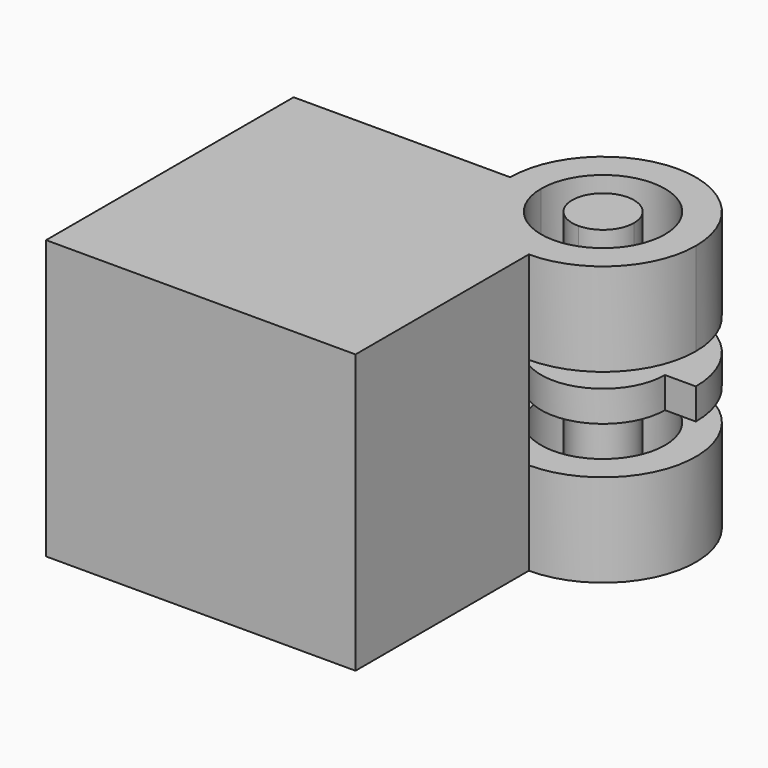
from build123d import *

# Parameters (mm, degrees)
F1_DEPTH  = 3
F2_DEPTH  = 1
F3_DEPTH  = 1
F5_DEPTH  = 1
F6_DEPTH  = 1
F8_DEPTH  = 1
F7_R      = 1
F9_DEPTH  = 1
F11_DEPTH = 3
F12_R     = 2
F13_DEPTH = 3
F14_DEPTH = 3


with BuildPart() as f1:
    # F0 (on Top) → F1 (new body)
    with BuildSketch(Plane.XY):
        with BuildLine():
            Line((-48.9987007827, 31.2983999767), (-55.9987007827, 31.2983999767))
            Line((-55.9987007827, 31.2983999767), (-55.9987007827, 21.2983999767))
            Line((-55.9987007827, 21.2983999767), (-45.9987007827, 21.2983999767))
            Line((-45.9987007827, 21.2983999767), (-45.9987007827, 28.2983999767))
            ThreePointArc((-45.9987007827, 28.2983999767), (-48.1200211262, 29.1770796331), (-48.9987007827, 31.2983999767))
        make_face()
        with BuildLine():
            ThreePointArc((-42.9987007827, 31.2983999767), (-45.9987007827, 34.2983999767), (-48.9987007827, 31.2983999767))
            Line((-48.9987007827, 31.2983999767), (-47.9987007827, 31.2983999767))
            ThreePointArc((-47.9987007827, 31.2983999767), (-45.9987007827, 33.2983999767), (-43.9987007827, 31.2983999767))
            ThreePointArc((-43.9987007827, 31.2983999767), (-44.5844872203, 29.8841864143), (-45.9987007827, 29.2983999767))
            Line((-45.9987007827, 29.2983999767), (-45.9987007827, 28.2983999767))
            ThreePointArc((-45.9987007827, 28.2983999767), (-43.8773804391, 29.1770796331), (-42.9987007827, 31.2983999767))
        make_face()
        with BuildLine():
            Line((-47.9987007827, 31.2983999767), (-48.9987007827, 31.2983999767))
            ThreePointArc((-48.9987007827, 31.2983999767), (-48.1200211262, 29.1770796331), (-45.9987007827, 28.2983999767))
            Line((-45.9987007827, 28.2983999767), (-45.9987007827, 29.2983999767))
            ThreePointArc((-45.9987007827, 29.2983999767), (-47.412914345, 29.8841864143), (-47.9987007827, 31.2983999767))
        make_face()
    extrude(amount=F1_DEPTH)

    # F0 (on Top) → F2 (join)
    with BuildSketch(Plane.XY):
        with BuildLine():
            Line((-48.9987007827, 31.2983999767), (-55.9987007827, 31.2983999767))
            Line((-55.9987007827, 31.2983999767), (-55.9987007827, 21.2983999767))
            Line((-55.9987007827, 21.2983999767), (-45.9987007827, 21.2983999767))
            Line((-45.9987007827, 21.2983999767), (-45.9987007827, 28.2983999767))
            ThreePointArc((-45.9987007827, 28.2983999767), (-48.1200211262, 29.1770796331), (-48.9987007827, 31.2983999767))
        make_face()
    extrude(amount=-F2_DEPTH)

    # F4 (on face) → F5 (join)
    with BuildSketch(Plane(origin=(0, 0, -1), x_dir=(1, 0, 0), z_dir=(0, 0, -1))):
        with BuildLine():
            ThreePointArc((-48.9987007827, -31.2983999767), (-48.1200211262, -29.1770796331), (-45.9987007827, -28.2983999767))
            Line((-45.9987007827, -28.2983999767), (-45.9987007827, -21.2983999767))
            Line((-45.9987007827, -21.2983999767), (-55.9987007827, -21.2983999767))
            Line((-55.9987007827, -21.2983999767), (-55.9987007827, -31.2983999767))
            Line((-55.9987007827, -31.2983999767), (-48.9987007827, -31.2983999767))
        make_face()
    extrude(amount=F5_DEPTH)

    # F7 (on face) → F8 (join)
    with BuildSketch(Plane(origin=(0, 0, -2), x_dir=(1, 0, 0), z_dir=(0, 0, -1))):
        with BuildLine():
            Line((-55.9987007827, -31.2983999767), (-48.9987007827, -31.2983999767))
            ThreePointArc((-48.9987007827, -31.2983999767), (-48.1200211262, -29.1770796331), (-45.9987007827, -28.2983999767))
            Line((-45.9987007827, -28.2983999767), (-45.9987007827, -21.2983999767))
            Line((-45.9987007827, -21.2983999767), (-55.9987007827, -21.2983999767))
            Line((-55.9987007827, -21.2983999767), (-55.9987007827, -31.2983999767))
        make_face()
    extrude(amount=F8_DEPTH)

    # F10 (on face) → F11 (join)
    with BuildSketch(Plane(origin=(0, 0, -3), x_dir=(1, 0, 0), z_dir=(0, 0, -1))):
        with BuildLine():
            Line((-55.9987007827, -21.2983999767), (-55.9987007827, -31.2983999767))
            Line((-55.9987007827, -31.2983999767), (-48.9987007827, -31.2983999767))
            ThreePointArc((-48.9987007827, -31.2983999767), (-48.1200211262, -29.1770796331), (-45.9987007827, -28.2983999767))
            Line((-45.9987007827, -28.2983999767), (-45.9987007827, -21.2983999767))
            Line((-45.9987007827, -21.2983999767), (-55.9987007827, -21.2983999767))
        make_face()
    extrude(amount=F11_DEPTH)

    # F12 (on face) → F13 (join, through all)
    with BuildSketch(Plane(origin=(0, 0, -3), x_dir=(1, 0, 0), z_dir=(0, 0, -1))):
        with BuildLine():
            ThreePointArc((-48.9987007827, -31.2983999767), (-43.8773804391, -33.4197203202), (-45.9987007827, -28.2983999767))
            ThreePointArc((-45.9987007827, -28.2983999767), (-48.1200211262, -29.1770796331), (-48.9987007827, -31.2983999767))
        make_face()
        with Locations((-45.9987007827, -31.2983999767)):
            Circle(F12_R, mode=Mode.SUBTRACT)
    extrude(amount=F13_DEPTH)


with BuildPart() as f1b:
    # F0 (on Top) → F1, piece 2 (new body)
    with BuildSketch(Plane.XY):
        with BuildLine():
            Line((-45.9987007827, 31.2983999767), (-46.9987007827, 31.2983999767))
            ThreePointArc((-46.9987007827, 31.2983999767), (-46.7058075638, 30.5912931955), (-45.9987007827, 30.2983999767))
            Line((-45.9987007827, 30.2983999767), (-45.9987007827, 31.2983999767))
        make_face()
        with BuildLine():
            ThreePointArc((-44.9987007827, 31.2983999767), (-45.9987007827, 32.2983999767), (-46.9987007827, 31.2983999767))
            Line((-46.9987007827, 31.2983999767), (-45.9987007827, 31.2983999767))
            Line((-45.9987007827, 31.2983999767), (-45.9987007827, 30.2983999767))
            ThreePointArc((-45.9987007827, 30.2983999767), (-45.2915940015, 30.5912931955), (-44.9987007827, 31.2983999767))
        make_face()
    extrude(amount=F1_DEPTH)

    # F0 (on Top) → F3 (join)
    with BuildSketch(Plane.XY):
        with BuildLine():
            Line((-45.9987007827, 31.2983999767), (-46.9987007827, 31.2983999767))
            ThreePointArc((-46.9987007827, 31.2983999767), (-46.7058075638, 30.5912931955), (-45.9987007827, 30.2983999767))
            Line((-45.9987007827, 30.2983999767), (-45.9987007827, 31.2983999767))
        make_face()
        with BuildLine():
            ThreePointArc((-44.9987007827, 31.2983999767), (-45.9987007827, 32.2983999767), (-46.9987007827, 31.2983999767))
            Line((-46.9987007827, 31.2983999767), (-45.9987007827, 31.2983999767))
            Line((-45.9987007827, 31.2983999767), (-45.9987007827, 30.2983999767))
            ThreePointArc((-45.9987007827, 30.2983999767), (-45.2915940015, 30.5912931955), (-44.9987007827, 31.2983999767))
        make_face()
    extrude(amount=-F3_DEPTH)

    # F4 (on face) → F6 (join)
    with BuildSketch(Plane(origin=(0, 0, -1), x_dir=(1, 0, 0), z_dir=(0, 0, -1))):
        with BuildLine():
            Line((-45.9987007827, -31.2983999767), (-44.9987007827, -31.2983999767))
            ThreePointArc((-44.9987007827, -31.2983999767), (-46.7058075638, -30.5912931955), (-45.9987007827, -32.2983999767))
            Line((-45.9987007827, -32.2983999767), (-45.9987007827, -31.2983999767))
        make_face()
        with BuildLine():
            Line((-44.9987007827, -31.2983999767), (-43.9987007827, -31.2983999767))
            ThreePointArc((-43.9987007827, -31.2983999767), (-47.412914345, -29.8841864143), (-45.9987007827, -33.2983999767))
            Line((-45.9987007827, -33.2983999767), (-45.9987007827, -32.2983999767))
            ThreePointArc((-45.9987007827, -32.2983999767), (-46.7058075638, -30.5912931955), (-44.9987007827, -31.2983999767))
        make_face()
        with BuildLine():
            ThreePointArc((-45.9987007827, -33.2983999767), (-44.5844872203, -32.712613539), (-43.9987007827, -31.2983999767))
            Line((-43.9987007827, -31.2983999767), (-44.9987007827, -31.2983999767))
            ThreePointArc((-44.9987007827, -31.2983999767), (-45.2915940015, -32.0055067579), (-45.9987007827, -32.2983999767))
            Line((-45.9987007827, -32.2983999767), (-45.9987007827, -33.2983999767))
        make_face()
        with BuildLine():
            ThreePointArc((-45.9987007827, -34.2983999767), (-43.8773804391, -33.4197203202), (-42.9987007827, -31.2983999767))
            Line((-42.9987007827, -31.2983999767), (-43.9987007827, -31.2983999767))
            ThreePointArc((-43.9987007827, -31.2983999767), (-44.5844872203, -32.712613539), (-45.9987007827, -33.2983999767))
            Line((-45.9987007827, -33.2983999767), (-45.9987007827, -34.2983999767))
        make_face()
        with BuildLine():
            ThreePointArc((-45.9987007827, -32.2983999767), (-45.2915940015, -32.0055067579), (-44.9987007827, -31.2983999767))
            Line((-44.9987007827, -31.2983999767), (-45.9987007827, -31.2983999767))
            Line((-45.9987007827, -31.2983999767), (-45.9987007827, -32.2983999767))
        make_face()
    extrude(amount=F6_DEPTH)

    # F7 (on face) → F9 (join)
    with BuildSketch(Plane(origin=(0, 0, -2), x_dir=(1, 0, 0), z_dir=(0, 0, -1))):
        with Locations((-45.9987007827, -31.2983999767)):
            Circle(F7_R)
    extrude(amount=F9_DEPTH)

    # F14 (add, through all): a face of the model
    f14_faces = [f1b.faces().sort_by_distance(p)[0] for p in [
        (-45.9987007827, 31.2983999767, -3),
    ]]
    extrude(f14_faces, amount=F14_DEPTH)


solid = Compound([f1.part, f1b.part])
